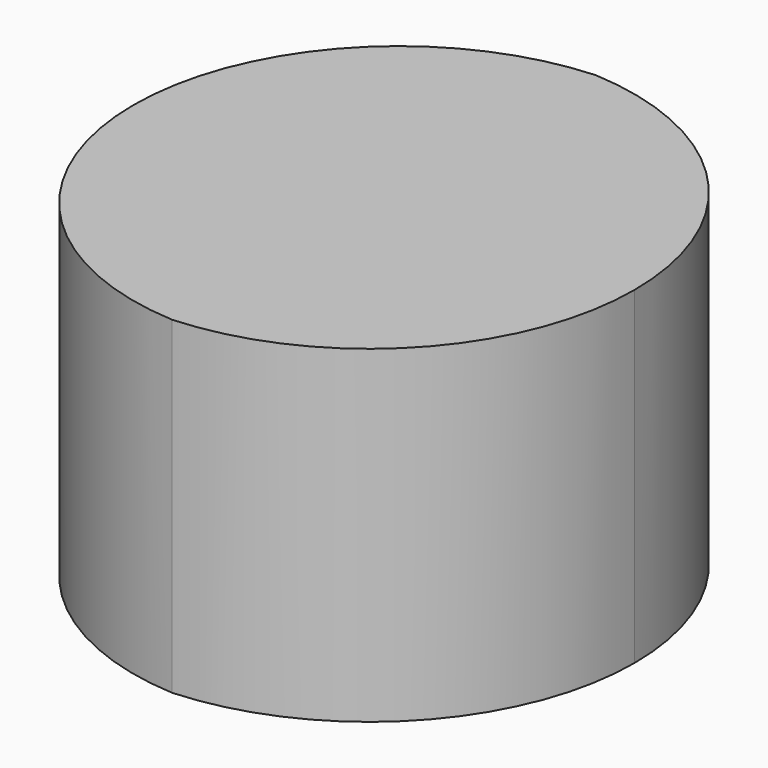
from build123d import *

# Parameters (mm, degrees)
F1_DEPTH    = 12.7
F2_T1_DEPTH = 79.2269835472


# Not quite as in the source:
# - a fillet or chamfer that OpenCascade refuses, or shapes differently, is made with other operations: its cross-section is extruded or revolved along the edge and cut away or added


with BuildPart() as f1:
    # F0 (on Front) → F1 (new body, symmetric)
    with BuildSketch(Plane.XZ):
        with BuildLine():
            Line((-11.0308257863, -15.9663576633), (-11.1952358857, -13.2855195552))
            Line((-11.1952358857, -13.2855195552), (-12.4416537583, -13.2855195552))
            Line((-12.4416537583, -13.2855195552), (-12.4416537583, -29.0125031024))
            Line((-12.4416537583, -29.0125031024), (-10.6407525752, -29.0125031024))
            Line((-10.6407525752, -29.0125031024), (9.3370480284, -29.0125031024))
            add(Edge.make_bspline(
                [(9.3370480284, -29.0125031024), (8.8163951875, -28.4602374533), (6.8919466336, -26.193166533), (5.7612829832, -22.5123911909), (7.5665201167, -17.4691949236), (8.3953980002, -15.9663576633)],
                knots=[0.9445205559, 0.9445205559, 0.9445205559, 0.9445205559, 0.9518406139, 0.9740303489, 0.9871444865, 0.9871444865, 0.9871444865, 0.9871444865], degree=3))
            Line((8.3953980003, -15.9663576633), (-11.0308257863, -15.9663576633))
        make_face()
        with BuildLine():
            Line((11.5424795076, -13.2855195552), (11.0820746049, -13.2855195552))
            Line((11.0820746049, -13.2855195552), (11.0820746049, -15.9663576633))
            Line((11.0820746049, -15.9663576633), (8.3953980003, -15.9663576633))
            add(Edge.make_bspline(
                [(9.3370480284, -29.0125031024), (8.8163951875, -28.4602374533), (6.8919466336, -26.193166533), (5.7612829832, -22.5123911909), (7.5665201167, -17.4691949236), (8.3953980002, -15.9663576633)],
                knots=[0.9445205559, 0.9445205559, 0.9445205559, 0.9445205559, 0.9518406139, 0.9740303489, 0.9871444865, 0.9871444865, 0.9871444865, 0.9871444865], degree=3))
            Line((9.3370480284, -29.0125031024), (10.6407525752, -29.0125031024))
            Line((10.6407525752, -29.0125031024), (11.5424795076, -29.0125031024))
            Line((11.5424795076, -29.0125031024), (11.5424795076, -13.2855195552))
        make_face()
        with BuildLine():
            Line((11.0820746049, -15.9663576633), (11.0820746049, -13.2855195552))
            Line((11.0820746049, -13.2855195552), (10.8409429303, -13.2855195552))
            add(Edge.make_bspline(
                [(8.3953980002, -15.9663576633), (9.1364610409, -14.6227373643), (10.004055933, -13.5752960653), (10.8409429303, -13.2855195552)],
                knots=[0.9871444865, 0.9871444865, 0.9871444865, 0.9871444865, 0.9988692567, 0.9988692567, 0.9988692567, 0.9988692567], degree=3))
            Line((8.3953980003, -15.9663576633), (11.0820746049, -15.9663576633))
        make_face()
        with BuildLine():
            add(Edge.make_bspline(
                [(8.3953980002, -15.9663576633), (9.1364610409, -14.6227373643), (10.004055933, -13.5752960653), (10.8409429303, -13.2855195552)],
                knots=[0.9871444865, 0.9871444865, 0.9871444865, 0.9871444865, 0.9988692567, 0.9988692567, 0.9988692567, 0.9988692567], degree=3))
            Line((10.8409429303, -13.2855195552), (-11.1952358857, -13.2855195552))
            Line((-11.1952358857, -13.2855195552), (-11.0308257863, -15.9663576633))
            Line((-11.0308257863, -15.9663576633), (8.3953980003, -15.9663576633))
        make_face()
    extrude(amount=F1_DEPTH, both=True)

    # F2: fillet of radius 12.7 on 4 edges, made by hand

    # F2_s2 → F2_t1 (cut)
    with BuildSketch(Plane.XY.offset(-60.7625031024)):
        with BuildLine():
            ThreePointArc((11.5424795076, 0), (7.8227356287, 8.9802561211), (-1.1575204924, 12.7))
            Line((-1.1575204924, 12.7), (11.5424795076, 12.7))
            Line((11.5424795076, 12.7), (11.5424795076, 0))
        make_face()
        with BuildLine():
            ThreePointArc((-12.4416537583, 0), (-8.7219098794, 8.9802561211), (0.2583462417, 12.7))
            Line((0.2583462417, 12.7), (-12.4416537583, 12.7))
            Line((-12.4416537583, 12.7), (-12.4416537583, 0))
        make_face()
        with BuildLine():
            ThreePointArc((-12.4416537583, 0), (-8.7219098794, -8.9802561211), (0.2583462417, -12.7))
            Line((0.2583462417, -12.7), (-12.4416537583, -12.7))
            Line((-12.4416537583, -12.7), (-12.4416537583, 0))
        make_face()
        with BuildLine():
            ThreePointArc((11.5424795076, 0), (7.8227356287, -8.9802561211), (-1.1575204924, -12.7))
            Line((-1.1575204924, -12.7), (11.5424795076, -12.7))
            Line((11.5424795076, -12.7), (11.5424795076, 0))
        make_face()
    extrude(amount=F2_T1_DEPTH, mode=Mode.SUBTRACT)


solid = f1.part
